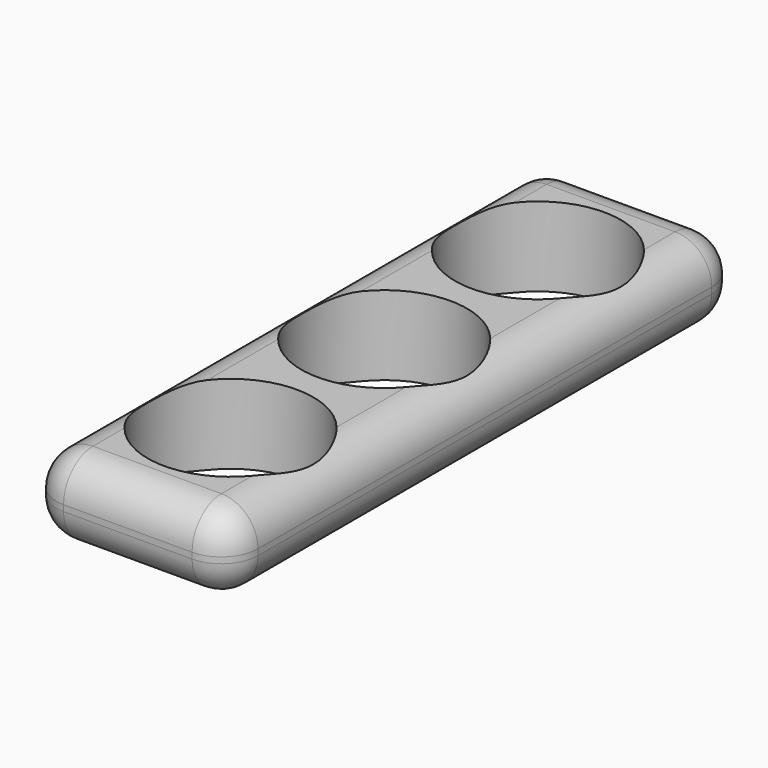
from build123d import *

# Parameters (mm, degrees)
F0_W         = 28
F0_H         = 88.9
F0_R         = 11.5
F1_DEPTH     = 11
F2_T1_DEPTH  = 78.74
F2_T3_DEPTH  = 17.84
F2_T5_DEPTH  = 0.84
F2_S9_W      = 5.08
F2_S9_H      = 5.08
F2_T10_DEPTH = 5.08
F2_S15_W     = 5.08
F2_S15_H     = 5.08
F2_T16_DEPTH = 5.08
F2_S21_W     = 5.08
F2_S21_H     = 5.08
F2_T22_DEPTH = 5.08
F2_S27_W     = 5.08
F2_S27_H     = 5.08
F2_T28_DEPTH = 5.08
F2_S33_W     = 5.08
F2_S33_H     = 5.08
F2_T34_DEPTH = 5.08
F2_S39_W     = 5.08
F2_S39_H     = 5.08
F2_T40_DEPTH = 5.08
F2_S45_W     = 5.08
F2_S45_H     = 5.08
F2_T46_DEPTH = 5.08
F2_S51_W     = 5.08
F2_S51_H     = 5.08
F2_T52_DEPTH = 5.08


# Not quite as in the source:
# - a fillet or chamfer that OpenCascade refuses, or shapes differently, is made with other operations: its cross-section is extruded or revolved along the edge and cut away or added


with BuildPart() as f1:
    # F0 (on Top) → F1 (new body)
    with BuildSketch(Plane.XY):
        with Locations((-14, 0)):
            Rectangle(F0_W, F0_H)
        with Locations((-13.97, -26.67)):
            Circle(F0_R, mode=Mode.SUBTRACT)
        with Locations((-13.97, 0)):
            Circle(F0_R, mode=Mode.SUBTRACT)
        with Locations((-13.97, 26.67)):
            Circle(F0_R, mode=Mode.SUBTRACT)
    extrude(amount=F1_DEPTH)

    # F2: fillet of radius 5.08 on 12 edges, made by hand

    # F2_s2 → F2_t1 (cut)
    with BuildSketch(Plane.XZ.offset(-39.37)):
        with BuildLine():
            ThreePointArc((0, 5.92), (-1.4878975516, 9.5121024484), (-5.08, 11))
            Line((-5.08, 11), (0, 11))
            Line((0, 11), (0, 5.92))
        make_face()
        with BuildLine():
            ThreePointArc((0, 5.08), (-1.4878975516, 1.4878975516), (-5.08, 0))
            Line((-5.08, 0), (0, 0))
            Line((0, 0), (0, 5.08))
        make_face()
        with BuildLine():
            ThreePointArc((-28, 5.92), (-26.5121024484, 9.5121024484), (-22.92, 11))
            Line((-22.92, 11), (-28, 11))
            Line((-28, 11), (-28, 5.92))
        make_face()
        with BuildLine():
            ThreePointArc((-28, 5.08), (-26.5121024484, 1.4878975516), (-22.92, 0))
            Line((-22.92, 0), (-28, 0))
            Line((-28, 0), (-28, 5.08))
        make_face()
    extrude(amount=F2_T1_DEPTH, mode=Mode.SUBTRACT)

    # F2_s4 → F2_t3 (cut)
    with BuildSketch(Plane.YZ.offset(-22.92)):
        with BuildLine():
            ThreePointArc((-44.45, 5.92), (-42.9621024484, 9.5121024484), (-39.37, 11))
            Line((-39.37, 11), (-44.45, 11))
            Line((-44.45, 11), (-44.45, 5.92))
        make_face()
        with BuildLine():
            ThreePointArc((-44.45, 5.08), (-42.9621024484, 1.4878975516), (-39.37, 0))
            Line((-39.37, 0), (-44.45, 0))
            Line((-44.45, 0), (-44.45, 5.08))
        make_face()
        with BuildLine():
            ThreePointArc((44.45, 5.92), (42.9621024484, 9.5121024484), (39.37, 11))
            Line((39.37, 11), (44.45, 11))
            Line((44.45, 11), (44.45, 5.92))
        make_face()
        with BuildLine():
            ThreePointArc((44.45, 5.08), (42.9621024484, 1.4878975516), (39.37, 0))
            Line((39.37, 0), (44.45, 0))
            Line((44.45, 0), (44.45, 5.08))
        make_face()
    extrude(amount=F2_T3_DEPTH, mode=Mode.SUBTRACT)

    # F2_s6 → F2_t5 (cut)
    with BuildSketch(Plane.XY.offset(5.08)):
        with BuildLine():
            ThreePointArc((0, -39.37), (-1.4878975516, -42.9621024484), (-5.08, -44.45))
            Line((-5.08, -44.45), (0, -44.45))
            Line((0, -44.45), (0, -39.37))
        make_face()
        with BuildLine():
            ThreePointArc((-28, -39.37), (-26.5121024484, -42.9621024484), (-22.92, -44.45))
            Line((-22.92, -44.45), (-28, -44.45))
            Line((-28, -44.45), (-28, -39.37))
        make_face()
        with BuildLine():
            ThreePointArc((-22.92, 44.45), (-26.5121024484, 42.9621024484), (-28, 39.37))
            Line((-28, 39.37), (-28, 44.45))
            Line((-28, 44.45), (-22.92, 44.45))
        make_face()
        with BuildLine():
            ThreePointArc((0, 39.37), (-1.4878975516, 42.9621024484), (-5.08, 44.45))
            Line((-5.08, 44.45), (0, 44.45))
            Line((0, 44.45), (0, 39.37))
        make_face()
    extrude(amount=F2_T5_DEPTH, mode=Mode.SUBTRACT)


with BuildPart() as f2_tool8:
    # F2_s9 → F2_t10 (new body)
    with BuildSketch(Plane.YZ.offset(-5.08)):
        with Locations((-41.91, 8.46)):
            Rectangle(F2_S9_W, F2_S9_H)
    extrude(amount=F2_T10_DEPTH)

    # F2_s11 → F2_t12 (revolve, cut)
    with BuildSketch(Plane(origin=(-5.08, -39.37, 5.92), x_dir=(0, 0.7071067812, -0.7071067812), z_dir=(0, -0.7071067812, -0.7071067812))):
        with BuildLine():
            ThreePointArc((0, -5.08), (5.08, 0), (0, 5.08))
            Line((0, 5.08), (0, -5.08))
        make_face()
    revolve(axis=Axis((-5.08, -39.37, 5.92), (1, 0, 0)), mode=Mode.SUBTRACT)


with BuildPart() as f1_1:
    add(f1.part)

    # F2_t7: cut F2_tool8
    add(f2_tool8.part, mode=Mode.SUBTRACT)


with BuildPart() as f2_tool14:
    # F2_s15 → F2_t16 (new body)
    with BuildSketch(Plane.YZ.offset(-5.08)):
        with Locations((41.91, 8.46)):
            Rectangle(F2_S15_W, F2_S15_H)
    extrude(amount=F2_T16_DEPTH)

    # F2_s17 → F2_t18 (revolve, cut)
    with BuildSketch(Plane(origin=(-5.08, 39.37, 5.92), x_dir=(0, -0.7071067812, -0.7071067812), z_dir=(0, -0.7071067812, 0.7071067812))):
        with BuildLine():
            ThreePointArc((0, -5.08), (5.08, 0), (0, 5.08))
            Line((0, 5.08), (0, -5.08))
        make_face()
    revolve(axis=Axis((-5.08, 39.37, 5.92), (1, 0, 0)), mode=Mode.SUBTRACT)


with BuildPart() as f1_2:
    add(f1_1.part)

    # F2_t13: cut F2_tool14
    add(f2_tool14.part, mode=Mode.SUBTRACT)


with BuildPart() as f2_tool20:
    # F2_s21 → F2_t22 (new body)
    with BuildSketch(Plane.XY.offset(5.92)):
        with Locations((-25.46, -41.91)):
            Rectangle(F2_S21_W, F2_S21_H)
    extrude(amount=F2_T22_DEPTH)

    # F2_s23 → F2_t24 (revolve, cut)
    with BuildSketch(Plane(origin=(-22.92, -39.37, 5.92), x_dir=(0.7071067812, 0.7071067812, 0), z_dir=(0.7071067812, -0.7071067812, 0))):
        with BuildLine():
            ThreePointArc((0, -5.08), (5.08, 0), (0, 5.08))
            Line((0, 5.08), (0, -5.08))
        make_face()
    revolve(axis=Axis((-22.92, -39.37, 5.92), (0, 0, 1)), mode=Mode.SUBTRACT)


with BuildPart() as f1_3:
    add(f1_2.part)

    # F2_t19: cut F2_tool20
    add(f2_tool20.part, mode=Mode.SUBTRACT)


with BuildPart() as f2_tool26:
    # F2_s27 → F2_t28 (new body)
    with BuildSketch(Plane.YZ.offset(-22.92)):
        with Locations((-41.91, 2.54)):
            Rectangle(F2_S27_W, F2_S27_H)
    extrude(amount=-F2_T28_DEPTH)

    # F2_s29 → F2_t30 (revolve, cut)
    with BuildSketch(Plane(origin=(-22.92, -39.37, 5.08), x_dir=(0, 0.7071067812, 0.7071067812), z_dir=(0, -0.7071067812, 0.7071067812))):
        with BuildLine():
            ThreePointArc((0, -5.08), (5.08, 0), (0, 5.08))
            Line((0, 5.08), (0, -5.08))
        make_face()
    revolve(axis=Axis((-22.92, -39.37, 5.08), (-1, 0, 0)), mode=Mode.SUBTRACT)


with BuildPart() as f1_4:
    add(f1_3.part)

    # F2_t25: cut F2_tool26
    add(f2_tool26.part, mode=Mode.SUBTRACT)


with BuildPart() as f2_tool32:
    # F2_s33 → F2_t34 (new body)
    with BuildSketch(Plane.YZ.offset(-5.08)):
        with Locations((-41.91, 2.54)):
            Rectangle(F2_S33_W, F2_S33_H)
    extrude(amount=F2_T34_DEPTH)

    # F2_s35 → F2_t36 (revolve, cut)
    with BuildSketch(Plane(origin=(-5.08, -39.37, 5.08), x_dir=(0, 0.7071067812, 0.7071067812), z_dir=(0, 0.7071067812, -0.7071067812))):
        with BuildLine():
            ThreePointArc((0, -5.08), (5.08, 0), (0, 5.08))
            Line((0, 5.08), (0, -5.08))
        make_face()
    revolve(axis=Axis((-5.08, -39.37, 5.08), (1, 0, 0)), mode=Mode.SUBTRACT)


with BuildPart() as f1_5:
    add(f1_4.part)

    # F2_t31: cut F2_tool32
    add(f2_tool32.part, mode=Mode.SUBTRACT)


with BuildPart() as f2_tool38:
    # F2_s39 → F2_t40 (new body)
    with BuildSketch(Plane.YZ.offset(-5.08)):
        with Locations((41.91, 2.54)):
            Rectangle(F2_S39_W, F2_S39_H)
    extrude(amount=F2_T40_DEPTH)

    # F2_s41 → F2_t42 (revolve, cut)
    with BuildSketch(Plane(origin=(-5.08, 39.37, 5.08), x_dir=(0, -0.7071067812, 0.7071067812), z_dir=(0, 0.7071067812, 0.7071067812))):
        with BuildLine():
            ThreePointArc((0, -5.08), (5.08, 0), (0, 5.08))
            Line((0, 5.08), (0, -5.08))
        make_face()
    revolve(axis=Axis((-5.08, 39.37, 5.08), (1, 0, 0)), mode=Mode.SUBTRACT)


with BuildPart() as f1_6:
    add(f1_5.part)

    # F2_t37: cut F2_tool38
    add(f2_tool38.part, mode=Mode.SUBTRACT)


with BuildPart() as f2_tool44:
    # F2_s45 → F2_t46 (new body)
    with BuildSketch(Plane.XY.offset(5.92)):
        with Locations((-25.46, 41.91)):
            Rectangle(F2_S45_W, F2_S45_H)
    extrude(amount=F2_T46_DEPTH)

    # F2_s47 → F2_t48 (revolve, cut)
    with BuildSketch(Plane(origin=(-22.92, 39.37, 5.92), x_dir=(0.7071067812, -0.7071067812, 0), z_dir=(-0.7071067812, -0.7071067812, 0))):
        with BuildLine():
            ThreePointArc((0, -5.08), (5.08, 0), (0, 5.08))
            Line((0, 5.08), (0, -5.08))
        make_face()
    revolve(axis=Axis((-22.92, 39.37, 5.92), (0, 0, 1)), mode=Mode.SUBTRACT)


with BuildPart() as f1_7:
    add(f1_6.part)

    # F2_t43: cut F2_tool44
    add(f2_tool44.part, mode=Mode.SUBTRACT)


with BuildPart() as f2_tool50:
    # F2_s51 → F2_t52 (new body)
    with BuildSketch(Plane.XZ.offset(-39.37)):
        with Locations((-25.46, 2.54)):
            Rectangle(F2_S51_W, F2_S51_H)
    extrude(amount=-F2_T52_DEPTH)

    # F2_s53 → F2_t54 (revolve, cut)
    with BuildSketch(Plane(origin=(-22.92, 39.37, 5.08), x_dir=(0.7071067812, 0, 0.7071067812), z_dir=(-0.7071067812, 0, 0.7071067812))):
        with BuildLine():
            ThreePointArc((0, -5.08), (5.08, 0), (0, 5.08))
            Line((0, 5.08), (0, -5.08))
        make_face()
    revolve(axis=Axis((-22.92, 39.37, 5.08), (0, 1, 0)), mode=Mode.SUBTRACT)


with BuildPart() as f1_8:
    add(f1_7.part)

    # F2_t49: cut F2_tool50
    add(f2_tool50.part, mode=Mode.SUBTRACT)


solid = f1_8.part
